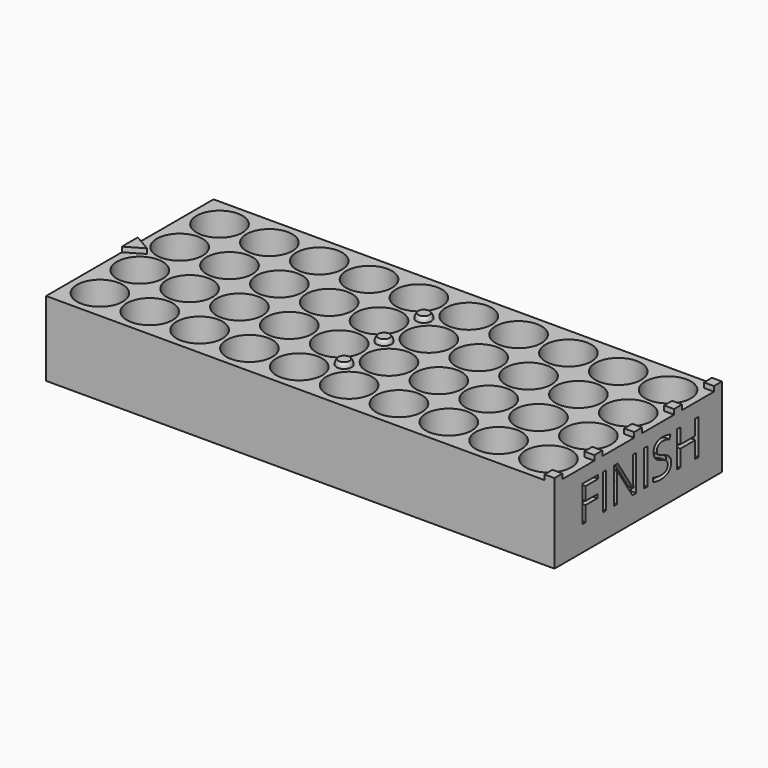
from build123d import *

# Parameters (mm, degrees)
F0_W         = 42
F0_H         = 102
F0_R         = 4.6
F1_DEPTH     = 15
F2_W         = 42
F2_H         = 2
F3_DEPTH     = 102
F5_ANGLE     = 180
F6_TEXT_SIZE = 11.2119183457
F7_DEPTH     = 1
F8_TEXT_SIZE = 9.990847889
F9_DEPTH     = 1
F10_W        = 2
F10_H        = 2
F11_DEPTH    = 1
F12_R        = 4.5
F13_R        = 1.5
F14_DEPTH    = 0.501
F15_ANGLE    = 90


# Not quite as in the source:
# - Text() gives the source's letters only with a copy of the font that has no kerning and outlines rounded to 1/6400 em; it was checked with that copy


with BuildPart() as f1:
    # F0 (on Top) → F1 (new body)
    with BuildSketch(Plane.XY):
        with Locations((-15, 45)):
            Rectangle(F0_W, F0_H)
        with Locations((-30, 0)):
            Circle(F0_R, mode=Mode.SUBTRACT)
        with Locations((-30, 10)):
            Circle(F0_R, mode=Mode.SUBTRACT)
        with Locations((-20, 0)):
            Circle(F0_R, mode=Mode.SUBTRACT)
        with Locations((-20, 10)):
            Circle(F0_R, mode=Mode.SUBTRACT)
        with Locations((-30, 20)):
            Circle(F0_R, mode=Mode.SUBTRACT)
        with Locations((-30, 30)):
            Circle(F0_R, mode=Mode.SUBTRACT)
        with Locations((-30, 40)):
            Circle(F0_R, mode=Mode.SUBTRACT)
        with Locations((-20, 20)):
            Circle(F0_R, mode=Mode.SUBTRACT)
        with Locations((-20, 30)):
            Circle(F0_R, mode=Mode.SUBTRACT)
        with Locations((-20, 40)):
            Circle(F0_R, mode=Mode.SUBTRACT)
        with Locations((-10, 0)):
            Circle(F0_R, mode=Mode.SUBTRACT)
        with Locations((-10, 10)):
            Circle(F0_R, mode=Mode.SUBTRACT)
        Circle(F0_R, mode=Mode.SUBTRACT)
        with Locations((0, 10)):
            Circle(F0_R, mode=Mode.SUBTRACT)
        with Locations((-10, 20)):
            Circle(F0_R, mode=Mode.SUBTRACT)
        with Locations((-10, 30)):
            Circle(F0_R, mode=Mode.SUBTRACT)
        with Locations((-10, 40)):
            Circle(F0_R, mode=Mode.SUBTRACT)
        with Locations((0, 20)):
            Circle(F0_R, mode=Mode.SUBTRACT)
        with Locations((0, 30)):
            Circle(F0_R, mode=Mode.SUBTRACT)
        with Locations((0, 40)):
            Circle(F0_R, mode=Mode.SUBTRACT)
        with Locations((-30, 50)):
            Circle(F0_R, mode=Mode.SUBTRACT)
        with Locations((-30, 60)):
            Circle(F0_R, mode=Mode.SUBTRACT)
        with Locations((-30, 70)):
            Circle(F0_R, mode=Mode.SUBTRACT)
        with Locations((-20, 50)):
            Circle(F0_R, mode=Mode.SUBTRACT)
        with Locations((-20, 60)):
            Circle(F0_R, mode=Mode.SUBTRACT)
        with Locations((-20, 70)):
            Circle(F0_R, mode=Mode.SUBTRACT)
        with Locations((-30, 80)):
            Circle(F0_R, mode=Mode.SUBTRACT)
        with Locations((-30, 90)):
            Circle(F0_R, mode=Mode.SUBTRACT)
        with Locations((-20, 80)):
            Circle(F0_R, mode=Mode.SUBTRACT)
        with Locations((-20, 90)):
            Circle(F0_R, mode=Mode.SUBTRACT)
        with Locations((-10, 50)):
            Circle(F0_R, mode=Mode.SUBTRACT)
        with Locations((-10, 60)):
            Circle(F0_R, mode=Mode.SUBTRACT)
        with Locations((-10, 70)):
            Circle(F0_R, mode=Mode.SUBTRACT)
        with Locations((0, 50)):
            Circle(F0_R, mode=Mode.SUBTRACT)
        with Locations((0, 60)):
            Circle(F0_R, mode=Mode.SUBTRACT)
        with Locations((0, 70)):
            Circle(F0_R, mode=Mode.SUBTRACT)
        with Locations((-10, 80)):
            Circle(F0_R, mode=Mode.SUBTRACT)
        with Locations((-10, 90)):
            Circle(F0_R, mode=Mode.SUBTRACT)
        with Locations((0, 80)):
            Circle(F0_R, mode=Mode.SUBTRACT)
        with Locations((0, 90)):
            Circle(F0_R, mode=Mode.SUBTRACT)
    extrude(amount=F1_DEPTH)

    # F2 (on face) → F3 (join)
    with BuildSketch(Plane.XZ.offset(6)):
        with Locations((-15, 1)):
            Rectangle(F2_W, F2_H)
    extrude(amount=-F3_DEPTH)

    # F4 (on face) → F5 (revolve)
    with BuildSketch(Plane.XY.offset(15)):
        with BuildLine():
            ThreePointArc((-13.5, 45), (-15, 46.5), (-16.5, 45))
            Line((-16.5, 45), (-13.5, 45))
        make_face()
        with BuildLine():
            ThreePointArc((-23.5, 45), (-25, 46.5), (-26.5, 45))
            Line((-26.5, 45), (-23.5, 45))
        make_face()
        with BuildLine():
            Line((-6.5, 45), (-3.5, 45))
            ThreePointArc((-3.5, 45), (-5, 46.5), (-6.5, 45))
        make_face()
    revolve(axis=Axis((-15, 45, 15), (1, 0, 0)), revolution_arc=F5_ANGLE)

    # F6 (on face) → F7 (cut)
    with BuildSketch(Plane.XZ.offset(6)):
        with Locations((-32.4812778198, 3.5215700703)):
            Text('START', F6_TEXT_SIZE, font='Open Sans', text_align=(TextAlign.LEFT, TextAlign.BOTTOM))
    extrude(amount=-F7_DEPTH, mode=Mode.SUBTRACT)

    # F8 (on face) → F9 (cut)
    with BuildSketch(Plane(origin=(0, 96, 0), x_dir=(-1, 0, 0), z_dir=(0, 1, 0))):
        with Locations((0, 5.0100044444)):
            Text('FINISH', F8_TEXT_SIZE, font='Open Sans', text_align=(TextAlign.LEFT, TextAlign.BOTTOM))
    extrude(amount=-F9_DEPTH, mode=Mode.SUBTRACT)

    # F10 (on face) → F11 (join)
    with BuildSketch(Plane.XY.offset(15)):
        Polygon((-15, -2.5358983849), (-17, -6), (-13, -6), align=None)
        with Locations((-15, 95)):
            Rectangle(F10_W, F10_H)
        with Locations((-25, 95)):
            Rectangle(F10_W, F10_H)
        with Locations((-5, 95)):
            Rectangle(F10_W, F10_H)
        with Locations((5, 95)):
            Rectangle(F10_W, F10_H)
        with Locations((-35, 95)):
            Rectangle(F10_W, F10_H)
    extrude(amount=F11_DEPTH)

    # F12
    f12_edges = [f1.edges().sort_by_distance(p)[0] for p in [
        (-34.6, 0, 2),
        (-34.6, 10, 2),
        (-34.6, 20, 2),
        (-34.6, 30, 2),
        (-34.6, 40, 2),
        (-34.6, 50, 2),
        (-34.6, 60, 2),
        (-34.6, 70, 2),
        (-34.6, 80, 2),
        (-34.6, 90, 2),
        (-24.6, 0, 2),
        (-24.6, 10, 2),
        (-24.6, 20, 2),
        (-24.6, 30, 2),
        (-24.6, 40, 2),
        (-24.6, 50, 2),
        (-24.6, 60, 2),
        (-24.6, 70, 2),
        (-24.6, 80, 2),
        (-24.6, 90, 2),
        (-14.6, 0, 2),
        (-14.6, 10, 2),
        (-14.6, 20, 2),
        (-14.6, 30, 2),
        (-14.6, 40, 2),
        (-14.6, 50, 2),
        (-14.6, 60, 2),
        (-14.6, 70, 2),
        (-14.6, 80, 2),
        (-14.6, 90, 2),
        (-4.6, 0, 2),
        (-4.6, 10, 2),
        (-4.6, 20, 2),
        (-4.6, 30, 2),
        (-4.6, 40, 2),
        (-4.6, 50, 2),
        (-4.6, 60, 2),
        (-4.6, 70, 2),
        (-4.6, 80, 2),
        (-4.6, 90, 2),
    ]]
    fillet(f12_edges, radius=F12_R)

    # F13 (on face) → F14 (cut, through all)
    with BuildSketch(Plane.XY.offset(16)):
        with Locations((-15, 45)):
            Circle(F13_R)
        with Locations((-25, 45)):
            Circle(F13_R)
        with Locations((-5, 45)):
            Circle(F13_R)
    extrude(amount=F14_DEPTH, mode=Mode.SUBTRACT)


with BuildPart() as f1_1:
    # F15: moved
    add(f1.part.rotate(Axis((-36, -6, 7.5), (0, 0, -1)), F15_ANGLE))


with BuildPart() as f1_2:
    # F16: moved
    add(f1_1.part.moved(Location((0, 70, 0))))


solid = f1_2.part
